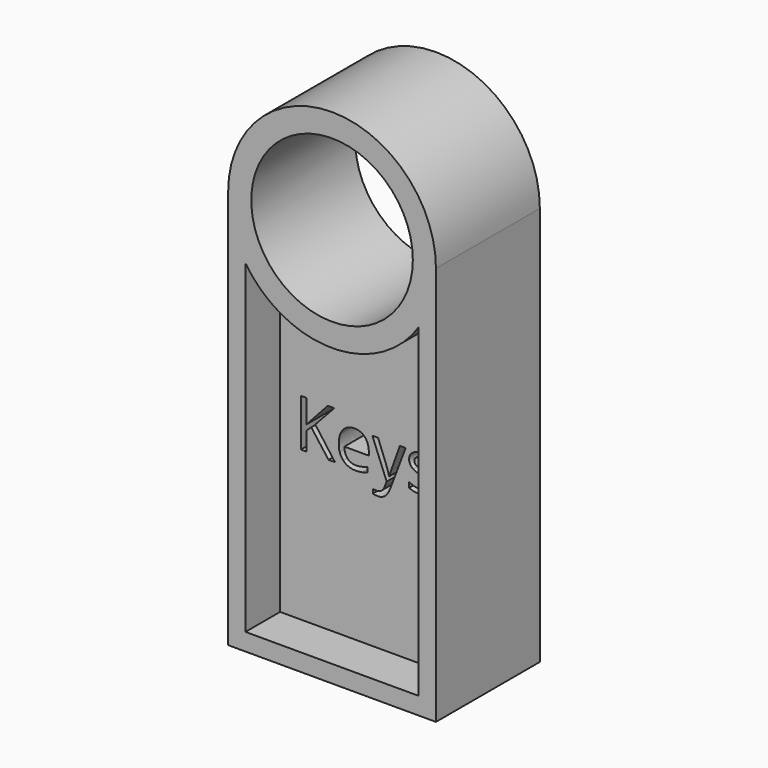
from build123d import *

# Parameters (mm, degrees)
F0_R     = 9.33
F1_DEPTH = 15
F2_DEPTH = 10


with BuildPart() as f1:
    # F0 (on Front) → F1 (new body)
    with BuildSketch(Plane.XZ):
        with BuildLine():
            ThreePointArc((-12.417365469, 39.4797180027), (-10.928240176, 42.6488659683), (-10.417365469, 46.1129675834))
            ThreePointArc((-10.417365469, 46.1129675834), (-22.417365469, 58.1129675834), (-34.417365469, 46.1129675834))
            ThreePointArc((-34.417365469, 46.1129675834), (-33.9064907621, 42.6488659683), (-32.417365469, 39.4797180027))
            ThreePointArc((-32.417365469, 39.4797180027), (-22.417365469, 34.1129675834), (-12.417365469, 39.4797180027))
        make_face()
        with Locations((-22.417365469, 46.1129675834)):
            Circle(F0_R, mode=Mode.SUBTRACT)
        with BuildLine():
            Line((-10.417365469, 0), (-10.417365469, 46.1129675834))
            ThreePointArc((-10.417365469, 46.1129675834), (-10.928240176, 42.6488659683), (-12.417365469, 39.4797180027))
            Line((-12.417365469, 39.4797180027), (-12.417365469, 2))
            Line((-12.417365469, 2), (-32.417365469, 2))
            Line((-32.417365469, 2), (-32.417365469, 39.4797180027))
            ThreePointArc((-32.417365469, 39.4797180027), (-33.9064907621, 42.6488659683), (-34.417365469, 46.1129675834))
            Line((-34.417365469, 46.1129675834), (-34.417365469, 0))
            Line((-34.417365469, 0), (-10.417365469, 0))
        make_face()
    extrude(amount=F1_DEPTH)

    # F0 (on Front) → F2 (join)
    with BuildSketch(Plane.XZ):
        with BuildLine():
            Line((-12.417365469, 2), (-12.417365469, 39.4797180027))
            ThreePointArc((-12.417365469, 39.4797180027), (-22.417365469, 34.1129675834), (-32.417365469, 39.4797180027))
            Line((-32.417365469, 39.4797180027), (-32.417365469, 2))
            Line((-32.417365469, 2), (-12.417365469, 2))
        make_face()
        with BuildLine():
            add(Edge.make_bspline(
                [(-22.9718386234, 19.2682127741), (-23.2651889221, 19.2059506699), (-23.6806687329, 19.2059506699)],
                knots=[0, 0, 0, 1, 1, 1], degree=2))
            add(Edge.make_bspline(
                [(-23.6806687329, 19.2059506699), (-24.5894559848, 19.2059506699), (-25.1156905003, 19.760322867)],
                knots=[0, 0, 0, 1, 1, 1], degree=2))
            add(Edge.make_bspline(
                [(-25.1156905003, 19.760322867), (-25.6419250157, 20.3146950642), (-25.6419250157, 21.2977179019)],
                knots=[0, 0, 0, 1, 1, 1], degree=2))
            add(Edge.make_bspline(
                [(-25.6419250157, 21.2977179019), (-25.6419250157, 22.2903195249), (-25.1534069672, 22.8740267519)],
                knots=[0, 0, 0, 1, 1, 1], degree=2))
            add(Edge.make_bspline(
                [(-25.1534069672, 22.8740267519), (-24.6648889188, 23.4577339789), (-23.8411133861, 23.4577339789)],
                knots=[0, 0, 0, 1, 1, 1], degree=2))
            add(Edge.make_bspline(
                [(-23.8411133861, 23.4577339789), (-23.0712185205, 23.4577339789), (-22.6222129612, 22.950657034)],
                knots=[0, 0, 0, 1, 1, 1], degree=2))
            add(Edge.make_bspline(
                [(-22.6222129612, 22.950657034), (-22.173207402, 22.4435800891), (-22.173207402, 21.6126204674)],
                knots=[0, 0, 0, 1, 1, 1], degree=2))
            Line((-22.173207402, 21.6126204674), (-22.173207402, 21.2198902716))
            Line((-22.173207402, 21.2198902716), (-24.9977517067, 21.2198902716))
            add(Edge.make_bspline(
                [(-24.9977517067, 21.2198902716), (-24.9785941362, 20.4978893323), (-24.6325605185, 20.123718033)],
                knots=[0, 0, 0, 1, 1, 1], degree=2))
            add(Edge.make_bspline(
                [(-24.6325605185, 20.123718033), (-24.2865269008, 19.7495467336), (-23.6579191179, 19.7495467336)],
                knots=[0, 0, 0, 1, 1, 1], degree=2))
            add(Edge.make_bspline(
                [(-23.6579191179, 19.7495467336), (-22.9957855865, 19.7495467336), (-22.3492175812, 20.0261341581)],
                knots=[0, 0, 0, 1, 1, 1], degree=2))
            Line((-22.3492175812, 20.0261341581), (-22.3492175812, 19.4717619609))
            add(Edge.make_bspline(
                [(-22.3492175812, 19.4717619609), (-22.6784883246, 19.3304748783), (-22.9718386234, 19.2682127741)],
                knots=[0, 0, 0, 1, 1, 1], degree=2))
        make_face(mode=Mode.SUBTRACT)
        Polygon((-28.3539185936, 22.3753312441), (-26.0717730044, 19.2813836038), (-26.8201156032, 19.2813836038), (-28.8137002863, 21.9347071219), (-29.3872300539, 21.4258341548), (-29.3872300539, 19.2813836038), (-30.0230219258, 19.2813836038), (-30.0230219258, 24.7520673377), (-29.3872300539, 24.7520673377), (-29.3872300539, 22.0388764117), (-26.9063246706, 24.7520673377), (-26.1543900273, 24.7520673377), align=None, mode=Mode.SUBTRACT)
        with BuildLine():
            Line((-20.1101765257, 19.2586339888), (-21.7649116801, 23.382301045))
            Line((-21.7649116801, 23.382301045), (-21.0979887561, 23.382301045))
            Line((-21.0979887561, 23.382301045), (-20.1999776376, 21.0438800924))
            add(Edge.make_bspline(
                [(-20.1999776376, 21.0438800924), (-19.9054299907, 20.2428541747), (-19.8335891012, 19.8872417718)],
                knots=[0, 0, 0, 1, 1, 1], degree=2))
            Line((-19.8335891012, 19.8872417718), (-19.8036553973, 19.8872417718))
            add(Edge.make_bspline(
                [(-19.8036553973, 19.8872417718), (-19.755761471, 20.078817477), (-19.6001062104, 20.540993866)],
                knots=[0, 0, 0, 1, 1, 1], degree=2))
            add(Edge.make_bspline(
                [(-19.6001062104, 20.540993866), (-19.4444509499, 21.003170255), (-18.5835576243, 23.382301045)],
                knots=[0, 0, 0, 1, 1, 1], degree=2))
            Line((-18.5835576243, 23.382301045), (-17.9178320484, 23.382301045))
            Line((-17.9178320484, 23.382301045), (-19.680328537, 18.7126432288))
            add(Edge.make_bspline(
                [(-19.680328537, 18.7126432288), (-19.9425477836, 18.0205759934), (-20.2921734457, 17.7302190651)],
                knots=[0, 0, 0, 1, 1, 1], degree=2))
            add(Edge.make_bspline(
                [(-20.2921734457, 17.7302190651), (-20.6417991079, 17.4398621368), (-21.150672075, 17.4398621368)],
                knots=[0, 0, 0, 1, 1, 1], degree=2))
            add(Edge.make_bspline(
                [(-21.150672075, 17.4398621368), (-21.4356409366, 17.4398621368), (-21.7122283611, 17.5045189373)],
                knots=[0, 0, 0, 1, 1, 1], degree=2))
            Line((-21.7122283611, 17.5045189373), (-21.7122283611, 18.0014184229))
            add(Edge.make_bspline(
                [(-21.7122283611, 18.0014184229), (-21.506284478, 17.9571165411), (-21.2524466685, 17.9571165411)],
                knots=[0, 0, 0, 1, 1, 1], degree=2))
            add(Edge.make_bspline(
                [(-21.2524466685, 17.9571165411), (-20.6118654039, 17.9571165411), (-20.3388700239, 18.6755254359)],
                knots=[0, 0, 0, 1, 1, 1], degree=2))
            Line((-20.3388700239, 18.6755254359), (-20.1101765257, 19.2586339888))
        make_face(mode=Mode.SUBTRACT)
        with BuildLine():
            add(Edge.make_bspline(
                [(-14.8633968974, 21.0774058408), (-14.6071643915, 20.8080025053), (-14.6071643915, 20.3997067834)],
                knots=[0, 0, 0, 1, 1, 1], degree=2))
            add(Edge.make_bspline(
                [(-14.6071643915, 20.3997067834), (-14.6071643915, 19.8273743639), (-15.0334203358, 19.5166625169)],
                knots=[0, 0, 0, 1, 1, 1], degree=2))
            add(Edge.make_bspline(
                [(-15.0334203358, 19.5166625169), (-15.45967628, 19.2059506699), (-16.2307684938, 19.2059506699)],
                knots=[0, 0, 0, 1, 1, 1], degree=2))
            add(Edge.make_bspline(
                [(-16.2307684938, 19.2059506699), (-17.0461625894, 19.2059506699), (-17.5023522376, 19.464577872)],
                knots=[0, 0, 0, 1, 1, 1], degree=2))
            Line((-17.5023522376, 19.464577872), (-17.5023522376, 20.040502336))
            add(Edge.make_bspline(
                [(-17.5023522376, 20.040502336), (-17.2066072426, 19.8908338162), (-16.8683563879, 19.8052234229)],
                knots=[0, 0, 0, 1, 1, 1], degree=2))
            add(Edge.make_bspline(
                [(-16.8683563879, 19.8052234229), (-16.5301055333, 19.7196130296), (-16.2152029677, 19.7196130296)],
                knots=[0, 0, 0, 1, 1, 1], degree=2))
            add(Edge.make_bspline(
                [(-16.2152029677, 19.7196130296), (-15.7290796156, 19.7196130296), (-15.4674590431, 19.8746696161)],
                knots=[0, 0, 0, 1, 1, 1], degree=2))
            add(Edge.make_bspline(
                [(-15.4674590431, 19.8746696161), (-15.2058384705, 20.0297262026), (-15.2058384705, 20.3482208126)],
                knots=[0, 0, 0, 1, 1, 1], degree=2))
            add(Edge.make_bspline(
                [(-15.2058384705, 20.3482208126), (-15.2058384705, 20.5876904442), (-15.4129797019, 20.7577138826)],
                knots=[0, 0, 0, 1, 1, 1], degree=2))
            add(Edge.make_bspline(
                [(-15.4129797019, 20.7577138826), (-15.6201209332, 20.9277373211), (-16.2235844048, 21.1600228637)],
                knots=[0, 0, 0, 1, 1, 1], degree=2))
            add(Edge.make_bspline(
                [(-16.2235844048, 21.1600228637), (-16.7959168244, 21.3731508358), (-17.0371824782, 21.5323981409)],
                knots=[0, 0, 0, 1, 1, 1], degree=2))
            add(Edge.make_bspline(
                [(-17.0371824782, 21.5323981409), (-17.278448132, 21.6916454459), (-17.3963869256, 21.8933986105)],
                knots=[0, 0, 0, 1, 1, 1], degree=2))
            add(Edge.make_bspline(
                [(-17.3963869256, 21.8933986105), (-17.5143257192, 22.0951517751), (-17.5143257192, 22.3753312441)],
                knots=[0, 0, 0, 1, 1, 1], degree=2))
            add(Edge.make_bspline(
                [(-17.5143257192, 22.3753312441), (-17.5143257192, 22.8770201223), (-17.1060299973, 23.1673770506)],
                knots=[0, 0, 0, 1, 1, 1], degree=2))
            add(Edge.make_bspline(
                [(-17.1060299973, 23.1673770506), (-16.6977342754, 23.4577339789), (-15.9877068177, 23.4577339789)],
                knots=[0, 0, 0, 1, 1, 1], degree=2))
            add(Edge.make_bspline(
                [(-15.9877068177, 23.4577339789), (-15.3255732863, 23.4577339789), (-14.6921761108, 23.1883306434)],
                knots=[0, 0, 0, 1, 1, 1], degree=2))
            Line((-14.6921761108, 23.1883306434), (-14.91368552, 22.6830497207))
            add(Edge.make_bspline(
                [(-14.91368552, 22.6830497207), (-15.5303198214, 22.9368875302), (-16.0320086996, 22.9368875302)],
                knots=[0, 0, 0, 1, 1, 1], degree=2))
            add(Edge.make_bspline(
                [(-16.0320086996, 22.9368875302), (-16.4738301699, 22.9368875302), (-16.6983329495, 22.7985938179)],
                knots=[0, 0, 0, 1, 1, 1], degree=2))
            add(Edge.make_bspline(
                [(-16.6983329495, 22.7985938179), (-16.9228357291, 22.6603001057), (-16.9228357291, 22.4172384296)],
                knots=[0, 0, 0, 1, 1, 1], degree=2))
            add(Edge.make_bspline(
                [(-16.9228357291, 22.4172384296), (-16.9228357291, 22.2520043838), (-16.838422684, 22.1364602866)],
                knots=[0, 0, 0, 1, 1, 1], degree=2))
            add(Edge.make_bspline(
                [(-16.838422684, 22.1364602866), (-16.7540096388, 22.0209161893), (-16.5672233262, 21.9161482255)],
                knots=[0, 0, 0, 1, 1, 1], degree=2))
            add(Edge.make_bspline(
                [(-16.5672233262, 21.9161482255), (-16.3804370135, 21.8113802617), (-15.8488144314, 21.6126204674)],
                knots=[0, 0, 0, 1, 1, 1], degree=2))
            add(Edge.make_bspline(
                [(-15.8488144314, 21.6126204674), (-15.1196294032, 21.3468091764), (-14.8633968974, 21.0774058408)],
                knots=[0, 0, 0, 1, 1, 1], degree=2))
        make_face(mode=Mode.SUBTRACT)
    extrude(amount=F2_DEPTH)


solid = f1.part
